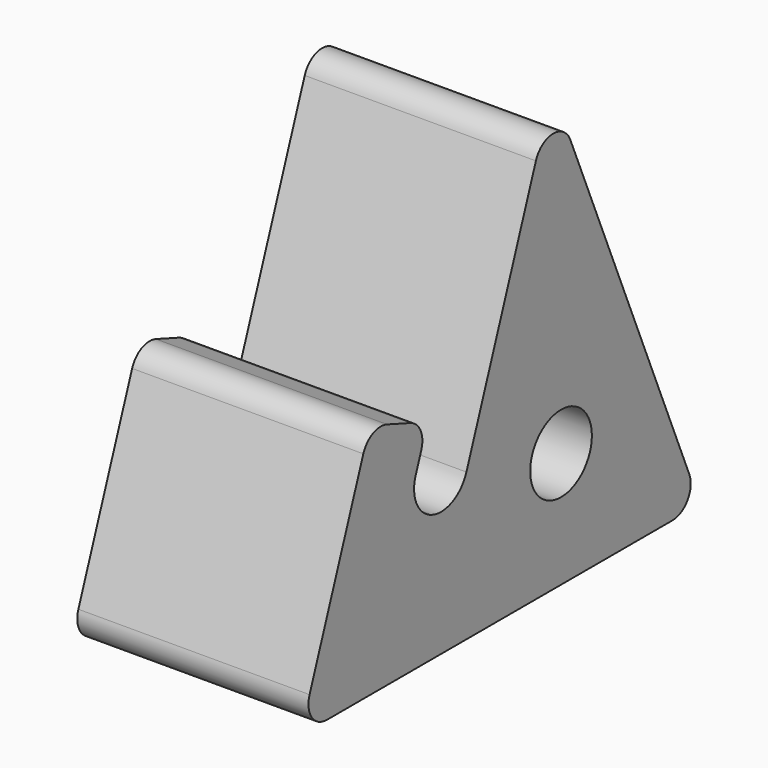
from build123d import *

# Parameters (mm, degrees)
F4_DEPTH = 30
F5_R     = 3
F6_R     = 5
F7_DEPTH = 33.1
F8_R     = 4.37499


# Not quite as in the source:
# - a fillet or chamfer is up to 0.001 mm smaller than in the source, because OpenCascade refuses the exact size


with BuildPart() as f4:
    # F3 (on Right) → F4 (new body)
    with BuildSketch(Plane.YZ):
        Polygon((-70.8067866115, 0), (-5.9983764602, 0), (-30.002993414, 57.2861679354), (-45.3938998636, 15), (-53.6162102955, 17.9926762541), (-50.1960088622, 27.389602462), (-59.5929350701, 30.8098038952), align=None)
    extrude(amount=F4_DEPTH)

    # F5
    f5_edges = [f4.edges().sort_by_distance(p)[0] for p in [
        (15, -50.196009, 27.389602),
        (15, -30.002993, 57.286168),
        (15, -59.592935, 30.809804),
        (15, -70.806787, 0),
        (15, -5.998376, 0),
    ]]
    fillet(f5_edges, radius=F5_R)

    # F6 (on face) → F7 (cut)
    with BuildSketch(Plane.YZ.offset(30)):
        with Locations((-28.5474918187, 15)):
            Circle(F6_R)
    extrude(amount=-F7_DEPTH, mode=Mode.SUBTRACT)

    # F8 (radius 4.375 in the source; OpenCascade refuses exactly that, so slightly less here)
    f8_edges = [f4.edges().sort_by_distance(p)[0] for p in [
        (15, -53.61621, 17.992676),
        (15, -45.3939, 15),
    ]]
    fillet(f8_edges, radius=F8_R)


solid = f4.part
